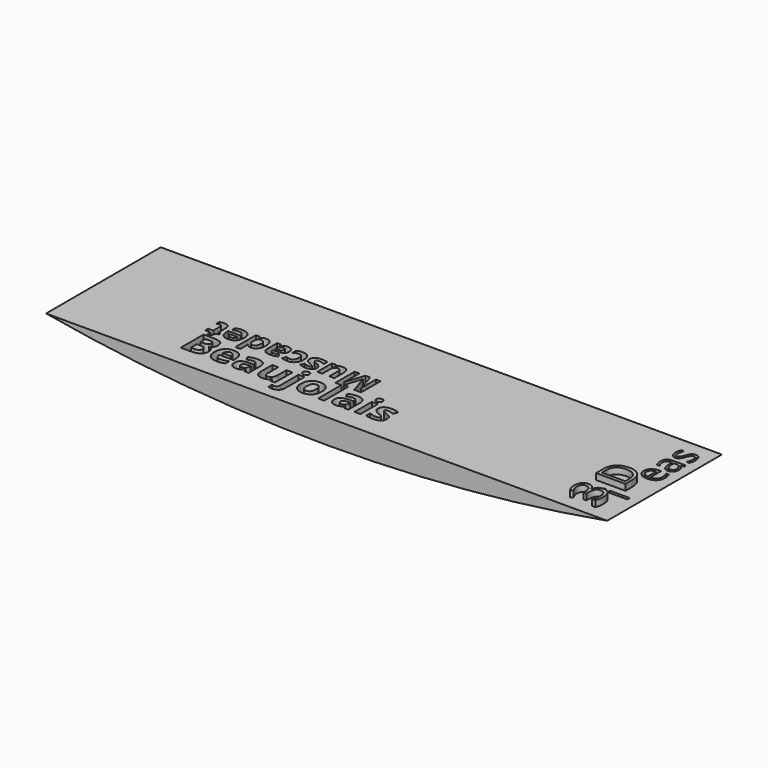
from build123d import *

# Parameters (mm, degrees)
F0_W         = 274
F0_H         = 70
F1_DEPTH     = 12
F2_TEXT_SIZE = 20.006252
F3_DEPTH     = 3
F4_TEXT_SIZE = 18.055556
F5_DEPTH     = 3
F7_DEPTH     = 70.001
F8_W         = 2.90735
F8_H         = 10.659264
F9_DEPTH     = 25


# Not quite as in the source:
# - Text() gives the source's letters only with a copy of the font that has no kerning and outlines rounded to 1/6400 em; it was checked with that copy


with BuildPart() as f1:
    # F0 (on Top) → F1 (new body)
    with BuildSketch(Plane.XY):
        Rectangle(F0_W, F0_H)
    extrude(amount=F1_DEPTH)

    # F2 (on face) → F3 (join)
    with BuildSketch(Plane.XY.offset(12)):
        with Locations(Location((127, -30), (0, 0, 90))):
            Text('3 D', F2_TEXT_SIZE, font='Open Sans', text_align=(TextAlign.LEFT, TextAlign.BOTTOM))
    extrude(amount=F3_DEPTH)

    # F4 (on face) → F5 (cut)
    with BuildSketch(Plane.XY.offset(12)):
        with Locations(Location((132, -18), (0, 0, 90))):
            Text('i   eas', F4_TEXT_SIZE, font='Open Sans', text_align=(TextAlign.LEFT, TextAlign.BOTTOM))
    extrude(amount=-F5_DEPTH, mode=Mode.SUBTRACT)

    # F6 (on face) → F7 (cut, through all)
    with BuildSketch(Plane.XZ.offset(35)):
        with BuildLine():
            ThreePointArc((0, 0), (-68.762272, 3.005732), (-137, 12))
            Line((-137, 12), (-137, 0))
            Line((-137, 0), (0, 0))
        make_face()
        with BuildLine():
            ThreePointArc((137, 12), (68.762272, 3.005732), (0, 0))
            Line((0, 0), (137, 0))
            Line((137, 0), (137, 12))
        make_face()
    extrude(amount=-F7_DEPTH, mode=Mode.SUBTRACT)

    # F8 (on face) → F9 (cut)
    with BuildSketch(Plane.XY.offset(12)):
        with BuildLine():
            Line((-74.907685, -11.061198), (-79.245828, -11.061198))
            Line((-79.245828, -11.061198), (-79.245828, -25))
            Line((-79.245828, -25), (-74.032124, -25))
            add(Edge.make_bspline(
                [(-70.288874, -23.932243), (-71.667806, -25), (-74.032124, -25)],
                knots=[0, 0, 0, 1, 1, 1], degree=2))
            add(Edge.make_bspline(
                [(-68.909942, -20.957778), (-68.909942, -22.864486), (-70.288874, -23.932243)],
                knots=[0, 0, 0, 1, 1, 1], degree=2))
            add(Edge.make_bspline(
                [(-69.497209, -18.802434), (-68.909942, -19.612404), (-68.909942, -20.957778)],
                knots=[0, 0, 0, 1, 1, 1], degree=2))
            add(Edge.make_bspline(
                [(-71.408493, -17.696544), (-70.084475, -17.992465), (-69.497209, -18.802434)],
                knots=[0, 0, 0, 1, 1, 1], degree=2))
            Line((-71.408493, -17.696544), (-71.408493, -17.601971))
            add(Edge.make_bspline(
                [(-69.849568, -16.639464), (-70.435309, -17.440282), (-71.408493, -17.601971)],
                knots=[0, 0, 0, 1, 1, 1], degree=2))
            add(Edge.make_bspline(
                [(-69.263827, -14.587846), (-69.263827, -15.838647), (-69.849568, -16.639464)],
                knots=[0, 0, 0, 1, 1, 1], degree=2))
            add(Edge.make_bspline(
                [(-70.6031, -11.904726), (-69.263827, -12.748253), (-69.263827, -14.587846)],
                knots=[0, 0, 0, 1, 1, 1], degree=2))
            add(Edge.make_bspline(
                [(-74.907685, -11.061198), (-71.942372, -11.061198), (-70.6031, -11.904726)],
                knots=[0, 0, 0, 1, 1, 1], degree=2))
        make_face()
        with BuildLine():
            Line((-76.289667, -22.559413), (-76.289667, -18.925989))
            Line((-76.289667, -18.925989), (-74.459227, -18.925989))
            add(Edge.make_bspline(
                [(-71.982031, -20.661857), (-71.982031, -18.925989), (-74.459227, -18.925989)],
                knots=[0, 0, 0, 1, 1, 1], degree=2))
            add(Edge.make_bspline(
                [(-72.563196, -22.092651), (-71.982031, -21.625889), (-71.982031, -20.661857)],
                knots=[0, 0, 0, 1, 1, 1], degree=2))
            add(Edge.make_bspline(
                [(-74.364654, -22.559413), (-73.144361, -22.559413), (-72.563196, -22.092651)],
                knots=[0, 0, 0, 1, 1, 1], degree=2))
            Line((-74.364654, -22.559413), (-76.289667, -22.559413))
        make_face(mode=Mode.SUBTRACT)
        with BuildLine():
            Line((-74.575155, -16.583026), (-76.289667, -16.583026))
            Line((-76.289667, -16.583026), (-76.289667, -13.48348))
            Line((-76.289667, -13.48348), (-74.736844, -13.48348))
            add(Edge.make_bspline(
                [(-72.881998, -13.831264), (-73.467738, -13.48348), (-74.736844, -13.48348)],
                knots=[0, 0, 0, 1, 1, 1], degree=2))
            add(Edge.make_bspline(
                [(-72.296257, -14.981391), (-72.296257, -14.179048), (-72.881998, -13.831264)],
                knots=[0, 0, 0, 1, 1, 1], degree=2))
            add(Edge.make_bspline(
                [(-72.834711, -16.210836), (-72.296257, -15.838647), (-72.296257, -14.981391)],
                knots=[0, 0, 0, 1, 1, 1], degree=2))
            add(Edge.make_bspline(
                [(-74.575155, -16.583026), (-73.373166, -16.583026), (-72.834711, -16.210836)],
                knots=[0, 0, 0, 1, 1, 1], degree=2))
        make_face(mode=Mode.SUBTRACT)
        with BuildLine():
            add(Edge.make_bspline(
                [(-61.533268, -25.192196), (-64.105037, -25.192196), (-65.554135, -23.770554)],
                knots=[0, 0, 0, 1, 1, 1], degree=2))
            add(Edge.make_bspline(
                [(-59.416059, -25.006101), (-60.282467, -25.192196), (-61.533268, -25.192196)],
                knots=[0, 0, 0, 1, 1, 1], degree=2))
            add(Edge.make_bspline(
                [(-57.786967, -24.438665), (-58.549651, -24.820007), (-59.416059, -25.006101)],
                knots=[0, 0, 0, 1, 1, 1], degree=2))
            Line((-57.786967, -24.438665), (-57.786967, -22.187224))
            add(Edge.make_bspline(
                [(-59.577748, -22.826352), (-58.720492, -22.626529), (-57.786967, -22.187224)],
                knots=[0, 0, 0, 1, 1, 1], degree=2))
            add(Edge.make_bspline(
                [(-61.399036, -23.026175), (-60.435004, -23.026175), (-59.577748, -22.826352)],
                knots=[0, 0, 0, 1, 1, 1], degree=2))
            add(Edge.make_bspline(
                [(-63.324049, -22.330608), (-62.637634, -23.026175), (-61.399036, -23.026175)],
                knots=[0, 0, 0, 1, 1, 1], degree=2))
            add(Edge.make_bspline(
                [(-64.059276, -20.396443), (-64.010464, -21.635041), (-63.324049, -22.330608)],
                knots=[0, 0, 0, 1, 1, 1], degree=2))
            Line((-64.059276, -20.396443), (-57.185973, -20.396443))
            Line((-57.185973, -20.396443), (-57.185973, -18.983953))
            add(Edge.make_bspline(
                [(-58.4444, -15.428323), (-57.185973, -16.714207), (-57.185973, -18.983953)],
                knots=[0, 0, 0, 1, 1, 1], degree=2))
            add(Edge.make_bspline(
                [(-61.960371, -14.142439), (-59.702828, -14.142439), (-58.4444, -15.428323)],
                knots=[0, 0, 0, 1, 1, 1], degree=2))
            add(Edge.make_bspline(
                [(-65.663962, -15.605266), (-64.32469, -14.142439), (-61.960371, -14.142439)],
                knots=[0, 0, 0, 1, 1, 1], degree=2))
            add(Edge.make_bspline(
                [(-67.003234, -19.746637), (-67.003234, -17.068092), (-65.663962, -15.605266)],
                knots=[0, 0, 0, 1, 1, 1], degree=2))
            add(Edge.make_bspline(
                [(-65.554135, -23.770554), (-67.003234, -22.348912), (-67.003234, -19.746637)],
                knots=[0, 0, 0, 1, 1, 1], degree=2))
        make_face()
        with BuildLine():
            add(Edge.make_bspline(
                [(-61.942067, -16.210836), (-62.866439, -16.210836), (-63.391165, -16.796577)],
                knots=[0, 0, 0, 1, 1, 1], degree=2))
            add(Edge.make_bspline(
                [(-60.474664, -16.796577), (-61.017694, -16.210836), (-61.942067, -16.210836)],
                knots=[0, 0, 0, 1, 1, 1], degree=2))
            add(Edge.make_bspline(
                [(-59.910278, -18.459227), (-59.931633, -17.382318), (-60.474664, -16.796577)],
                knots=[0, 0, 0, 1, 1, 1], degree=2))
            Line((-59.910278, -18.459227), (-63.99216, -18.459227))
            add(Edge.make_bspline(
                [(-63.391165, -16.796577), (-63.915891, -17.382318), (-63.99216, -18.459227)],
                knots=[0, 0, 0, 1, 1, 1], degree=2))
        make_face(mode=Mode.SUBTRACT)
        with BuildLine():
            Line((-48.616462, -23.550901), (-48.052076, -25))
            Line((-48.052076, -25), (-46.023338, -25))
            Line((-46.023338, -25), (-46.023338, -17.897892))
            add(Edge.make_bspline(
                [(-47.167363, -15.056134), (-46.023338, -15.991183), (-46.023338, -17.897892)],
                knots=[0, 0, 0, 1, 1, 1], degree=2))
            add(Edge.make_bspline(
                [(-50.456054, -14.121084), (-48.311388, -14.121084), (-47.167363, -15.056134)],
                knots=[0, 0, 0, 1, 1, 1], degree=2))
            add(Edge.make_bspline(
                [(-54.534885, -15.085115), (-52.695293, -14.121084), (-50.456054, -14.121084)],
                knots=[0, 0, 0, 1, 1, 1], degree=2))
            Line((-54.534885, -15.085115), (-53.573904, -17.049788))
            add(Edge.make_bspline(
                [(-50.568931, -16.277952), (-51.847189, -16.277952), (-53.573904, -17.049788)],
                knots=[0, 0, 0, 1, 1, 1], degree=2))
            add(Edge.make_bspline(
                [(-48.909332, -17.897892), (-48.909332, -16.277952), (-50.568931, -16.277952)],
                knots=[0, 0, 0, 1, 1, 1], degree=2))
            Line((-48.909332, -17.897892), (-48.909332, -18.364654))
            Line((-48.909332, -18.364654), (-50.761128, -18.422618))
            add(Edge.make_bspline(
                [(-54.339638, -19.313432), (-53.152903, -18.508039), (-50.761128, -18.422618)],
                knots=[0, 0, 0, 1, 1, 1], degree=2))
            add(Edge.make_bspline(
                [(-55.526374, -21.815034), (-55.526374, -20.118826), (-54.339638, -19.313432)],
                knots=[0, 0, 0, 1, 1, 1], degree=2))
            add(Edge.make_bspline(
                [(-54.644712, -24.313585), (-55.526374, -23.434974), (-55.526374, -21.815034)],
                knots=[0, 0, 0, 1, 1, 1], degree=2))
            add(Edge.make_bspline(
                [(-52.22853, -25.192196), (-53.76305, -25.192196), (-54.644712, -24.313585)],
                knots=[0, 0, 0, 1, 1, 1], degree=2))
            add(Edge.make_bspline(
                [(-50.202843, -24.833735), (-50.98078, -25.192196), (-52.22853, -25.192196)],
                knots=[0, 0, 0, 1, 1, 1], degree=2))
            add(Edge.make_bspline(
                [(-48.69273, -23.550901), (-49.424906, -24.475274), (-50.202843, -24.833735)],
                knots=[0, 0, 0, 1, 1, 1], degree=2))
            Line((-48.69273, -23.550901), (-48.616462, -23.550901))
        make_face()
        with BuildLine():
            Line((-50.035053, -20.100522), (-48.909332, -20.060862))
            Line((-48.909332, -20.060862), (-48.909332, -20.939473))
            add(Edge.make_bspline(
                [(-49.514903, -22.483145), (-48.909332, -21.900455), (-48.909332, -20.939473)],
                knots=[0, 0, 0, 1, 1, 1], degree=2))
            add(Edge.make_bspline(
                [(-51.133317, -23.065835), (-50.120473, -23.065835), (-49.514903, -22.483145)],
                knots=[0, 0, 0, 1, 1, 1], degree=2))
            add(Edge.make_bspline(
                [(-52.542756, -21.833338), (-52.542756, -23.065835), (-51.133317, -23.065835)],
                knots=[0, 0, 0, 1, 1, 1], degree=2))
            add(Edge.make_bspline(
                [(-51.923457, -20.556606), (-52.542756, -20.976082), (-52.542756, -21.833338)],
                knots=[0, 0, 0, 1, 1, 1], degree=2))
            add(Edge.make_bspline(
                [(-50.035053, -20.100522), (-51.304158, -20.13713), (-51.923457, -20.556606)],
                knots=[0, 0, 0, 1, 1, 1], degree=2))
        make_face(mode=Mode.SUBTRACT)
        with BuildLine():
            Line((-35.867446, -23.636322), (-35.476952, -25))
            Line((-35.476952, -25), (-33.246865, -25))
            Line((-33.246865, -25), (-33.246865, -14.340736))
            Line((-33.246865, -14.340736), (-36.154215, -14.340736))
            Line((-36.154215, -14.340736), (-36.154215, -19.356143))
            add(Edge.make_bspline(
                [(-36.697245, -22.059093), (-36.154215, -21.244547), (-36.154215, -19.356143)],
                knots=[0, 0, 0, 1, 1, 1], degree=2))
            add(Edge.make_bspline(
                [(-38.460569, -22.873639), (-37.240276, -22.873639), (-36.697245, -22.059093)],
                knots=[0, 0, 0, 1, 1, 1], degree=2))
            add(Edge.make_bspline(
                [(-39.767809, -22.29705), (-39.357485, -22.873639), (-38.460569, -22.873639)],
                knots=[0, 0, 0, 1, 1, 1], degree=2))
            add(Edge.make_bspline(
                [(-40.178132, -20.567284), (-40.178132, -21.720461), (-39.767809, -22.29705)],
                knots=[0, 0, 0, 1, 1, 1], degree=2))
            Line((-40.178132, -20.567284), (-40.178132, -14.340736))
            Line((-40.178132, -14.340736), (-43.085482, -14.340736))
            Line((-43.085482, -14.340736), (-43.085482, -21.290308))
            add(Edge.make_bspline(
                [(-42.132127, -24.185454), (-43.085482, -23.178712), (-43.085482, -21.290308)],
                knots=[0, 0, 0, 1, 1, 1], degree=2))
            add(Edge.make_bspline(
                [(-39.299521, -25.192196), (-41.178773, -25.192196), (-42.132127, -24.185454)],
                knots=[0, 0, 0, 1, 1, 1], degree=2))
            add(Edge.make_bspline(
                [(-37.345526, -24.786449), (-38.204308, -25.192196), (-39.299521, -25.192196)],
                knots=[0, 0, 0, 1, 1, 1], degree=2))
            add(Edge.make_bspline(
                [(-36.019982, -23.636322), (-36.486745, -24.380701), (-37.345526, -24.786449)],
                knots=[0, 0, 0, 1, 1, 1], degree=2))
            Line((-36.019982, -23.636322), (-35.867446, -23.636322))
        make_face()
        with BuildLine():
            add(Edge.make_bspline(
                [(-31.053388, -29.692028), (-32.169956, -29.692028), (-32.969249, -29.45102)],
                knots=[0, 0, 0, 1, 1, 1], degree=2))
            add(Edge.make_bspline(
                [(-28.271119, -28.770707), (-29.253455, -29.692028), (-31.053388, -29.692028)],
                knots=[0, 0, 0, 1, 1, 1], degree=2))
            add(Edge.make_bspline(
                [(-27.288782, -26.153177), (-27.288782, -27.849385), (-28.271119, -28.770707)],
                knots=[0, 0, 0, 1, 1, 1], degree=2))
            Line((-27.288782, -26.153177), (-27.288782, -14.340736))
            Line((-27.288782, -14.340736), (-30.196132, -14.340736))
            Line((-30.196132, -14.340736), (-30.196132, -25.726075))
            add(Edge.make_bspline(
                [(-30.534763, -26.935691), (-30.196132, -26.525367), (-30.196132, -25.726075)],
                knots=[0, 0, 0, 1, 1, 1], degree=2))
            add(Edge.make_bspline(
                [(-31.605571, -27.346014), (-30.873395, -27.346014), (-30.534763, -26.935691)],
                knots=[0, 0, 0, 1, 1, 1], degree=2))
            add(Edge.make_bspline(
                [(-32.969249, -27.16297), (-32.304189, -27.346014), (-31.605571, -27.346014)],
                knots=[0, 0, 0, 1, 1, 1], degree=2))
            Line((-32.969249, -27.16297), (-32.969249, -29.45102))
        make_face()
        with BuildLine():
            add(Edge.make_bspline(
                [(-30.321212, -11.585924), (-30.321212, -10.164282), (-28.737881, -10.164282)],
                knots=[0, 0, 0, 1, 1, 1], degree=2))
            add(Edge.make_bspline(
                [(-28.737881, -13.016718), (-30.321212, -13.016718), (-30.321212, -11.585924)],
                knots=[0, 0, 0, 1, 1, 1], degree=2))
            add(Edge.make_bspline(
                [(-27.54962, -12.639952), (-27.94469, -13.016718), (-28.737881, -13.016718)],
                knots=[0, 0, 0, 1, 1, 1], degree=2))
            add(Edge.make_bspline(
                [(-27.15455, -11.585924), (-27.15455, -12.263187), (-27.54962, -12.639952)],
                knots=[0, 0, 0, 1, 1, 1], degree=2))
            add(Edge.make_bspline(
                [(-28.737881, -10.164282), (-27.15455, -10.164282), (-27.15455, -11.585924)],
                knots=[0, 0, 0, 1, 1, 1], degree=2))
        make_face()
        with BuildLine():
            add(Edge.make_bspline(
                [(-14.551969, -19.652064), (-14.551969, -22.25434), (-15.924799, -23.723268)],
                knots=[0, 0, 0, 1, 1, 1], degree=2))
            add(Edge.make_bspline(
                [(-15.18042, -16.724885), (-14.551969, -17.97416), (-14.551969, -19.652064)],
                knots=[0, 0, 0, 1, 1, 1], degree=2))
            add(Edge.make_bspline(
                [(-16.981879, -14.809024), (-15.808872, -15.475609), (-15.18042, -16.724885)],
                knots=[0, 0, 0, 1, 1, 1], degree=2))
            add(Edge.make_bspline(
                [(-19.689405, -14.142439), (-18.154886, -14.142439), (-16.981879, -14.809024)],
                knots=[0, 0, 0, 1, 1, 1], degree=2))
            add(Edge.make_bspline(
                [(-23.522652, -15.591537), (-22.160499, -14.142439), (-19.689405, -14.142439)],
                knots=[0, 0, 0, 1, 1, 1], degree=2))
            add(Edge.make_bspline(
                [(-24.884804, -19.652064), (-24.884804, -17.040636), (-23.522652, -15.591537)],
                knots=[0, 0, 0, 1, 1, 1], degree=2))
            add(Edge.make_bspline(
                [(-24.256353, -22.588395), (-24.884804, -21.329967), (-24.884804, -19.652064)],
                knots=[0, 0, 0, 1, 1, 1], degree=2))
            add(Edge.make_bspline(
                [(-22.454895, -24.519509), (-23.627902, -23.846823), (-24.256353, -22.588395)],
                knots=[0, 0, 0, 1, 1, 1], degree=2))
            add(Edge.make_bspline(
                [(-19.747369, -25.192196), (-21.281888, -25.192196), (-22.454895, -24.519509)],
                knots=[0, 0, 0, 1, 1, 1], degree=2))
            add(Edge.make_bspline(
                [(-15.924799, -23.723268), (-17.29763, -25.192196), (-19.747369, -25.192196)],
                knots=[0, 0, 0, 1, 1, 1], degree=2))
        make_face()
        with BuildLine():
            add(Edge.make_bspline(
                [(-21.922542, -19.652064), (-21.922542, -21.235395), (-21.402392, -22.045364)],
                knots=[0, 0, 0, 1, 1, 1], degree=2))
            add(Edge.make_bspline(
                [(-21.406968, -17.272492), (-21.922542, -18.059581), (-21.922542, -19.652064)],
                knots=[0, 0, 0, 1, 1, 1], degree=2))
            add(Edge.make_bspline(
                [(-19.729064, -16.485402), (-20.891394, -16.485402), (-21.406968, -17.272492)],
                knots=[0, 0, 0, 1, 1, 1], degree=2))
            add(Edge.make_bspline(
                [(-18.040483, -17.277068), (-18.554532, -16.485402), (-19.729064, -16.485402)],
                knots=[0, 0, 0, 1, 1, 1], degree=2))
            add(Edge.make_bspline(
                [(-17.526435, -19.652064), (-17.526435, -18.068733), (-18.040483, -17.277068)],
                knots=[0, 0, 0, 1, 1, 1], degree=2))
            add(Edge.make_bspline(
                [(-18.035907, -22.049941), (-17.526435, -21.244547), (-17.526435, -19.652064)],
                knots=[0, 0, 0, 1, 1, 1], degree=2))
            add(Edge.make_bspline(
                [(-19.71076, -22.855334), (-18.54538, -22.855334), (-18.035907, -22.049941)],
                knots=[0, 0, 0, 1, 1, 1], degree=2))
            add(Edge.make_bspline(
                [(-21.402392, -22.045364), (-20.882242, -22.855334), (-19.71076, -22.855334)],
                knots=[0, 0, 0, 1, 1, 1], degree=2))
        make_face(mode=Mode.SUBTRACT)
        Polygon((-12.147991, -25), (-9.240642, -25), (-9.240642, -10.164282), (-11.470686, -10.164282), (-11.693005, -10.841512), (-12.147991, -10.841512), align=None)
        with BuildLine():
            Line((-15.096382, -10.841512), (-12.147991, -10.841512))
            Line((-12.147991, -10.841512), (-12.147991, -10.164282))
            Line((-12.147991, -10.164282), (-11.470686, -10.164282))
            Line((-11.470686, -10.164282), (-8.73119, -1.819208))
            Line((-8.73119, -1.819208), (-8.682128, -1.819208))
            Line((-8.682128, -1.819208), (-5.890739, -10.841512))
            Line((-5.890739, -10.841512), (-2.484781, -10.841512))
            Line((-2.484781, -10.841512), (-2.484781, 0.956687))
            Line((-2.484781, 0.956687), (-4.72099, 0.956687))
            Line((-4.72099, 0.956687), (-4.72099, -4.530547))
            add(Edge.make_bspline(
                [(-4.566057, -8.298018), (-4.72099, -5.475643), (-4.72099, -4.530547)],
                knots=[0, 0, 0, 1, 1, 1], degree=2))
            Line((-4.566057, -8.298018), (-4.638359, -8.298018))
            Line((-4.638359, -8.298018), (-7.47881, 0.956687))
            Line((-7.47881, 0.956687), (-9.771828, 0.956687))
            Line((-9.771828, 0.956687), (-12.813692, -8.282524))
            Line((-12.813692, -8.282524), (-12.885995, -8.282524))
            add(Edge.make_bspline(
                [(-12.777541, -5.540199), (-12.790452, -6.056644), (-12.885995, -8.282524)],
                knots=[0, 0, 0, 1, 1, 1], degree=2))
            add(Edge.make_bspline(
                [(-12.76463, -4.628672), (-12.76463, -5.023753), (-12.777541, -5.540199)],
                knots=[0, 0, 0, 1, 1, 1], degree=2))
            Line((-12.76463, -4.628672), (-12.76463, 0.956687))
            Line((-12.76463, 0.956687), (-15.096382, 0.956687))
            Line((-15.096382, 0.956687), (-15.096382, -10.841512))
        make_face()
        Polygon((-12.147991, -10.164282), (-12.147991, -10.841512), (-11.693005, -10.841512), (-11.470686, -10.164282), align=None)
        with BuildLine():
            Line((0.015284, -23.550901), (0.57967, -25))
            Line((0.57967, -25), (2.608408, -25))
            Line((2.608408, -25), (2.608408, -17.897892))
            add(Edge.make_bspline(
                [(1.464383, -15.056134), (2.608408, -15.991183), (2.608408, -17.897892)],
                knots=[0, 0, 0, 1, 1, 1], degree=2))
            add(Edge.make_bspline(
                [(-1.824308, -14.121084), (0.320358, -14.121084), (1.464383, -15.056134)],
                knots=[0, 0, 0, 1, 1, 1], degree=2))
            add(Edge.make_bspline(
                [(-5.903139, -15.085115), (-4.063547, -14.121084), (-1.824308, -14.121084)],
                knots=[0, 0, 0, 1, 1, 1], degree=2))
            Line((-5.903139, -15.085115), (-4.942158, -17.049788))
            add(Edge.make_bspline(
                [(-1.937185, -16.277952), (-3.215443, -16.277952), (-4.942158, -17.049788)],
                knots=[0, 0, 0, 1, 1, 1], degree=2))
            add(Edge.make_bspline(
                [(-0.277586, -17.897892), (-0.277586, -16.277952), (-1.937185, -16.277952)],
                knots=[0, 0, 0, 1, 1, 1], degree=2))
            Line((-0.277586, -17.897892), (-0.277586, -18.364654))
            Line((-0.277586, -18.364654), (-2.129382, -18.422618))
            add(Edge.make_bspline(
                [(-5.707892, -19.313432), (-4.521157, -18.508039), (-2.129382, -18.422618)],
                knots=[0, 0, 0, 1, 1, 1], degree=2))
            add(Edge.make_bspline(
                [(-6.894628, -21.815034), (-6.894628, -20.118826), (-5.707892, -19.313432)],
                knots=[0, 0, 0, 1, 1, 1], degree=2))
            add(Edge.make_bspline(
                [(-6.012966, -24.313585), (-6.894628, -23.434974), (-6.894628, -21.815034)],
                knots=[0, 0, 0, 1, 1, 1], degree=2))
            add(Edge.make_bspline(
                [(-3.596785, -25.192196), (-5.131304, -25.192196), (-6.012966, -24.313585)],
                knots=[0, 0, 0, 1, 1, 1], degree=2))
            add(Edge.make_bspline(
                [(-1.571097, -24.833735), (-2.349034, -25.192196), (-3.596785, -25.192196)],
                knots=[0, 0, 0, 1, 1, 1], degree=2))
            add(Edge.make_bspline(
                [(-0.060984, -23.550901), (-0.79316, -24.475274), (-1.571097, -24.833735)],
                knots=[0, 0, 0, 1, 1, 1], degree=2))
            Line((-0.060984, -23.550901), (0.015284, -23.550901))
        make_face()
        with BuildLine():
            Line((-1.403307, -20.100522), (-0.277586, -20.060862))
            Line((-0.277586, -20.060862), (-0.277586, -20.939473))
            add(Edge.make_bspline(
                [(-0.883157, -22.483145), (-0.277586, -21.900455), (-0.277586, -20.939473)],
                knots=[0, 0, 0, 1, 1, 1], degree=2))
            add(Edge.make_bspline(
                [(-2.501571, -23.065835), (-1.488728, -23.065835), (-0.883157, -22.483145)],
                knots=[0, 0, 0, 1, 1, 1], degree=2))
            add(Edge.make_bspline(
                [(-3.91101, -21.833338), (-3.91101, -23.065835), (-2.501571, -23.065835)],
                knots=[0, 0, 0, 1, 1, 1], degree=2))
            add(Edge.make_bspline(
                [(-3.291711, -20.556606), (-3.91101, -20.976082), (-3.91101, -21.833338)],
                knots=[0, 0, 0, 1, 1, 1], degree=2))
            add(Edge.make_bspline(
                [(-1.403307, -20.100522), (-2.672412, -20.13713), (-3.291711, -20.556606)],
                knots=[0, 0, 0, 1, 1, 1], degree=2))
        make_face(mode=Mode.SUBTRACT)
        with BuildLine():
            add(Edge.make_bspline(
                [(5.479148, -11.585924), (5.479148, -10.164282), (7.062479, -10.164282)],
                knots=[0, 0, 0, 1, 1, 1], degree=2))
            add(Edge.make_bspline(
                [(7.062479, -13.016718), (5.479148, -13.016718), (5.479148, -11.585924)],
                knots=[0, 0, 0, 1, 1, 1], degree=2))
            add(Edge.make_bspline(
                [(8.25074, -12.639952), (7.85567, -13.016718), (7.062479, -13.016718)],
                knots=[0, 0, 0, 1, 1, 1], degree=2))
            add(Edge.make_bspline(
                [(8.64581, -11.585924), (8.64581, -12.263187), (8.25074, -12.639952)],
                knots=[0, 0, 0, 1, 1, 1], degree=2))
            add(Edge.make_bspline(
                [(7.062479, -10.164282), (8.64581, -10.164282), (8.64581, -11.585924)],
                knots=[0, 0, 0, 1, 1, 1], degree=2))
        make_face()
        with Locations((7.057903, -19.670368)):
            Rectangle(F8_W, F8_H)
        with BuildLine():
            add(Edge.make_bspline(
                [(19, -21.833338), (19, -23.474633), (17.860551, -24.333415)],
                knots=[0, 0, 0, 1, 1, 1], degree=2))
            add(Edge.make_bspline(
                [(18.722383, -20.471186), (19, -21.043198), (19, -21.833338)],
                knots=[0, 0, 0, 1, 1, 1], degree=2))
            add(Edge.make_bspline(
                [(17.863602, -19.461393), (18.444766, -19.899173), (18.722383, -20.471186)],
                knots=[0, 0, 0, 1, 1, 1], degree=2))
            add(Edge.make_bspline(
                [(16.034687, -18.517191), (17.282437, -19.023613), (17.863602, -19.461393)],
                knots=[0, 0, 0, 1, 1, 1], degree=2))
            add(Edge.make_bspline(
                [(14.21645, -17.669087), (14.631349, -17.955856), (16.034687, -18.517191)],
                knots=[0, 0, 0, 1, 1, 1], degree=2))
            add(Edge.make_bspline(
                [(13.80155, -16.991824), (13.80155, -17.382318), (14.21645, -17.669087)],
                knots=[0, 0, 0, 1, 1, 1], degree=2))
            add(Edge.make_bspline(
                [(15.088959, -16.296257), (13.80155, -16.296257), (13.80155, -16.991824)],
                knots=[0, 0, 0, 1, 1, 1], degree=2))
            add(Edge.make_bspline(
                [(16.510601, -16.51591), (15.815034, -16.296257), (15.088959, -16.296257)],
                knots=[0, 0, 0, 1, 1, 1], degree=2))
            add(Edge.make_bspline(
                [(18.008512, -17.077245), (17.206169, -16.735562), (16.510601, -16.51591)],
                knots=[0, 0, 0, 1, 1, 1], degree=2))
            Line((18.008512, -17.077245), (18.884072, -14.981391))
            add(Edge.make_bspline(
                [(15.137771, -14.142439), (17.062784, -14.142439), (18.884072, -14.981391)],
                knots=[0, 0, 0, 1, 1, 1], degree=2))
            add(Edge.make_bspline(
                [(12.015345, -14.91885), (13.115135, -14.142439), (15.137771, -14.142439)],
                knots=[0, 0, 0, 1, 1, 1], degree=2))
            add(Edge.make_bspline(
                [(10.915556, -17.116904), (10.915556, -15.695262), (12.015345, -14.91885)],
                knots=[0, 0, 0, 1, 1, 1], degree=2))
            add(Edge.make_bspline(
                [(11.176393, -18.511089), (10.915556, -17.943653), (10.915556, -17.116904)],
                knots=[0, 0, 0, 1, 1, 1], degree=2))
            add(Edge.make_bspline(
                [(12.015345, -19.517832), (11.437231, -19.078526), (11.176393, -18.511089)],
                knots=[0, 0, 0, 1, 1, 1], degree=2))
            add(Edge.make_bspline(
                [(13.822905, -20.472711), (12.593459, -19.957137), (12.015345, -19.517832)],
                knots=[0, 0, 0, 1, 1, 1], degree=2))
            add(Edge.make_bspline(
                [(15.19421, -21.104213), (14.680161, -20.832698), (13.822905, -20.472711)],
                knots=[0, 0, 0, 1, 1, 1], degree=2))
            add(Edge.make_bspline(
                [(15.918759, -21.590805), (15.708258, -21.375728), (15.19421, -21.104213)],
                knots=[0, 0, 0, 1, 1, 1], degree=2))
            add(Edge.make_bspline(
                [(16.12926, -22.150615), (16.12926, -21.805882), (15.918759, -21.590805)],
                knots=[0, 0, 0, 1, 1, 1], degree=2))
            add(Edge.make_bspline(
                [(14.545929, -23.065835), (16.12926, -23.065835), (16.12926, -22.150615)],
                knots=[0, 0, 0, 1, 1, 1], degree=2))
            add(Edge.make_bspline(
                [(12.758199, -22.808048), (13.774093, -23.065835), (14.545929, -23.065835)],
                knots=[0, 0, 0, 1, 1, 1], degree=2))
            add(Edge.make_bspline(
                [(10.93386, -22.168919), (11.742305, -22.550261), (12.758199, -22.808048)],
                knots=[0, 0, 0, 1, 1, 1], degree=2))
            Line((10.93386, -22.168919), (10.93386, -24.569847))
            add(Edge.make_bspline(
                [(12.468379, -25.033558), (11.647732, -24.87492), (10.93386, -24.569847)],
                knots=[0, 0, 0, 1, 1, 1], degree=2))
            add(Edge.make_bspline(
                [(14.451356, -25.192196), (13.289027, -25.192196), (12.468379, -25.033558)],
                knots=[0, 0, 0, 1, 1, 1], degree=2))
            add(Edge.make_bspline(
                [(17.860551, -24.333415), (16.721102, -25.192196), (14.451356, -25.192196)],
                knots=[0, 0, 0, 1, 1, 1], degree=2))
        make_face()
        with BuildLine():
            Line((-23.932765, -0.197569), (-24.26329, 0.956687))
            Line((-24.26329, 0.956687), (-26.150899, 0.956687))
            Line((-26.150899, 0.956687), (-26.150899, -8.065617))
            Line((-26.150899, -8.065617), (-23.690036, -8.065617))
            Line((-23.690036, -8.065617), (-23.690036, -3.820435))
            add(Edge.make_bspline(
                [(-23.230399, -1.532581), (-23.690036, -2.222036), (-23.690036, -3.820435)],
                knots=[0, 0, 0, 1, 1, 1], degree=2))
            add(Edge.make_bspline(
                [(-21.737872, -0.843126), (-22.770763, -0.843126), (-23.230399, -1.532581)],
                knots=[0, 0, 0, 1, 1, 1], degree=2))
            add(Edge.make_bspline(
                [(-20.631387, -1.331167), (-20.978697, -0.843126), (-21.737872, -0.843126)],
                knots=[0, 0, 0, 1, 1, 1], degree=2))
            add(Edge.make_bspline(
                [(-20.284077, -2.79529), (-20.284077, -1.819208), (-20.631387, -1.331167)],
                knots=[0, 0, 0, 1, 1, 1], degree=2))
            Line((-20.284077, -2.79529), (-20.284077, -8.065617))
            Line((-20.284077, -8.065617), (-17.823214, -8.065617))
            Line((-17.823214, -8.065617), (-17.823214, -2.183302))
            add(Edge.make_bspline(
                [(-18.63016, 0.267232), (-17.823214, -0.584903), (-17.823214, -2.183302)],
                knots=[0, 0, 0, 1, 1, 1], degree=2))
            add(Edge.make_bspline(
                [(-21.027759, 1.119367), (-19.437107, 1.119367), (-18.63016, 0.267232)],
                knots=[0, 0, 0, 1, 1, 1], degree=2))
            add(Edge.make_bspline(
                [(-22.681676, 0.775931), (-21.954779, 1.119367), (-21.027759, 1.119367)],
                knots=[0, 0, 0, 1, 1, 1], degree=2))
            add(Edge.make_bspline(
                [(-23.803654, -0.197569), (-23.408573, 0.432494), (-22.681676, 0.775931)],
                knots=[0, 0, 0, 1, 1, 1], degree=2))
            Line((-23.803654, -0.197569), (-23.932765, -0.197569))
        make_face()
        with BuildLine():
            add(Edge.make_bspline(
                [(-35.028598, -1.723666), (-35.028598, -0.334427), (-34.064136, 0.39247)],
                knots=[0, 0, 0, 1, 1, 1], degree=2))
            add(Edge.make_bspline(
                [(-34.793615, -2.876631), (-35.028598, -2.392463), (-35.028598, -1.723666)],
                knots=[0, 0, 0, 1, 1, 1], degree=2))
            add(Edge.make_bspline(
                [(-34.066718, -3.731348), (-34.558633, -3.360798), (-34.793615, -2.876631)],
                knots=[0, 0, 0, 1, 1, 1], degree=2))
            add(Edge.make_bspline(
                [(-32.518673, -4.530547), (-33.574804, -4.101898), (-34.066718, -3.731348)],
                knots=[0, 0, 0, 1, 1, 1], degree=2))
            add(Edge.make_bspline(
                [(-30.979665, -5.248407), (-31.330848, -5.005677), (-32.518673, -4.530547)],
                knots=[0, 0, 0, 1, 1, 1], degree=2))
            add(Edge.make_bspline(
                [(-30.628482, -5.821661), (-30.628482, -5.491136), (-30.979665, -5.248407)],
                knots=[0, 0, 0, 1, 1, 1], degree=2))
            add(Edge.make_bspline(
                [(-31.718182, -6.410409), (-30.628482, -6.410409), (-30.628482, -5.821661)],
                knots=[0, 0, 0, 1, 1, 1], degree=2))
            add(Edge.make_bspline(
                [(-32.9215, -6.224489), (-32.332752, -6.410409), (-31.718182, -6.410409)],
                knots=[0, 0, 0, 1, 1, 1], degree=2))
            add(Edge.make_bspline(
                [(-34.189374, -5.749359), (-33.510248, -6.038568), (-32.9215, -6.224489)],
                knots=[0, 0, 0, 1, 1, 1], degree=2))
            Line((-34.189374, -5.749359), (-34.930474, -7.523349))
            add(Edge.make_bspline(
                [(-31.759498, -8.233462), (-33.388884, -8.233462), (-34.930474, -7.523349)],
                knots=[0, 0, 0, 1, 1, 1], degree=2))
            add(Edge.make_bspline(
                [(-29.116588, -7.576285), (-30.047481, -8.233462), (-31.759498, -8.233462)],
                knots=[0, 0, 0, 1, 1, 1], degree=2))
            add(Edge.make_bspline(
                [(-28.185694, -5.71579), (-28.185694, -6.919108), (-29.116588, -7.576285)],
                knots=[0, 0, 0, 1, 1, 1], degree=2))
            add(Edge.make_bspline(
                [(-28.406475, -4.535712), (-28.185694, -5.016006), (-28.185694, -5.71579)],
                knots=[0, 0, 0, 1, 1, 1], degree=2))
            add(Edge.make_bspline(
                [(-29.116588, -3.683577), (-28.627255, -4.055418), (-28.406475, -4.535712)],
                knots=[0, 0, 0, 1, 1, 1], degree=2))
            add(Edge.make_bspline(
                [(-30.646558, -2.875339), (-29.60592, -3.311736), (-29.116588, -3.683577)],
                knots=[0, 0, 0, 1, 1, 1], degree=2))
            add(Edge.make_bspline(
                [(-31.807269, -2.340818), (-31.372164, -2.570637), (-30.646558, -2.875339)],
                knots=[0, 0, 0, 1, 1, 1], degree=2))
            add(Edge.make_bspline(
                [(-32.420548, -1.928953), (-32.242374, -2.111), (-31.807269, -2.340818)],
                knots=[0, 0, 0, 1, 1, 1], degree=2))
            add(Edge.make_bspline(
                [(-32.598722, -1.455114), (-32.598722, -1.746906), (-32.420548, -1.928953)],
                knots=[0, 0, 0, 1, 1, 1], degree=2))
            add(Edge.make_bspline(
                [(-31.258546, -0.680446), (-32.598722, -0.680446), (-32.598722, -1.455114)],
                knots=[0, 0, 0, 1, 1, 1], degree=2))
            add(Edge.make_bspline(
                [(-29.74536, -0.898644), (-30.605242, -0.680446), (-31.258546, -0.680446)],
                knots=[0, 0, 0, 1, 1, 1], degree=2))
            add(Edge.make_bspline(
                [(-28.201188, -1.439621), (-28.885478, -1.116842), (-29.74536, -0.898644)],
                knots=[0, 0, 0, 1, 1, 1], degree=2))
            Line((-28.201188, -1.439621), (-28.201188, 0.592593))
            add(Edge.make_bspline(
                [(-29.500048, 0.985091), (-28.805429, 0.850815), (-28.201188, 0.592593)],
                knots=[0, 0, 0, 1, 1, 1], degree=2))
            add(Edge.make_bspline(
                [(-31.178496, 1.119367), (-30.194668, 1.119367), (-29.500048, 0.985091)],
                knots=[0, 0, 0, 1, 1, 1], degree=2))
            add(Edge.make_bspline(
                [(-34.064136, 0.39247), (-33.099674, 1.119367), (-31.178496, 1.119367)],
                knots=[0, 0, 0, 1, 1, 1], degree=2))
        make_face()
        with BuildLine():
            add(Edge.make_bspline(
                [(-40.611375, 1.119367), (-36.399761, 1.119367), (-36.399761, -3.505403)],
                knots=[0, 0, 0, 1, 1, 1], degree=2))
            add(Edge.make_bspline(
                [(-42.1478, 0.973471), (-41.538394, 1.119367), (-40.611375, 1.119367)],
                knots=[0, 0, 0, 1, 1, 1], degree=2))
            add(Edge.make_bspline(
                [(-43.353701, 0.447988), (-42.757206, 0.827575), (-42.1478, 0.973471)],
                knots=[0, 0, 0, 1, 1, 1], degree=2))
            Line((-43.353701, 0.447988), (-43.353701, -1.65911))
            add(Edge.make_bspline(
                [(-42.143927, -1.063907), (-42.749459, -1.2537), (-43.353701, -1.65911)],
                knots=[0, 0, 0, 1, 1, 1], degree=2))
            add(Edge.make_bspline(
                [(-40.828282, -0.874113), (-41.538394, -0.874113), (-42.143927, -1.063907)],
                knots=[0, 0, 0, 1, 1, 1], degree=2))
            add(Edge.make_bspline(
                [(-38.907104, -3.520896), (-38.907104, -0.874113), (-40.828282, -0.874113)],
                knots=[0, 0, 0, 1, 1, 1], degree=2))
            add(Edge.make_bspline(
                [(-40.828282, -6.250311), (-38.907104, -6.250311), (-38.907104, -3.520896)],
                knots=[0, 0, 0, 1, 1, 1], degree=2))
            add(Edge.make_bspline(
                [(-41.828895, -6.100542), (-41.329234, -6.250311), (-40.828282, -6.250311)],
                knots=[0, 0, 0, 1, 1, 1], degree=2))
            add(Edge.make_bspline(
                [(-42.909557, -5.71579), (-42.328556, -5.950773), (-41.828895, -6.100542)],
                knots=[0, 0, 0, 1, 1, 1], degree=2))
            Line((-42.909557, -5.71579), (-43.637746, -7.621474))
            add(Edge.make_bspline(
                [(-40.828282, -8.233462), (-42.393112, -8.233462), (-43.637746, -7.621474)],
                knots=[0, 0, 0, 1, 1, 1], degree=2))
            add(Edge.make_bspline(
                [(-37.544979, -7.019815), (-38.690197, -8.233462), (-40.828282, -8.233462)],
                knots=[0, 0, 0, 1, 1, 1], degree=2))
            add(Edge.make_bspline(
                [(-36.399761, -3.505403), (-36.399761, -5.806168), (-37.544979, -7.019815)],
                knots=[0, 0, 0, 1, 1, 1], degree=2))
        make_face()
        with BuildLine():
            Line((-50.697557, -0.269872), (-51.175269, 0.956687))
            Line((-51.175269, 0.956687), (-52.89245, 0.956687))
            Line((-52.89245, 0.956687), (-52.89245, -5.05474))
            add(Edge.make_bspline(
                [(-51.924115, -7.460085), (-52.89245, -6.668632), (-52.89245, -5.05474)],
                knots=[0, 0, 0, 1, 1, 1], degree=2))
            add(Edge.make_bspline(
                [(-49.140473, -8.251538), (-50.955779, -8.251538), (-51.924115, -7.460085)],
                knots=[0, 0, 0, 1, 1, 1], degree=2))
            add(Edge.make_bspline(
                [(-45.688035, -7.435554), (-47.245118, -8.251538), (-49.140473, -8.251538)],
                knots=[0, 0, 0, 1, 1, 1], degree=2))
            Line((-45.688035, -7.435554), (-46.501436, -5.772599))
            add(Edge.make_bspline(
                [(-49.044931, -6.425903), (-47.962977, -6.425903), (-46.501436, -5.772599)],
                knots=[0, 0, 0, 1, 1, 1], degree=2))
            add(Edge.make_bspline(
                [(-50.449663, -5.05474), (-50.449663, -6.425903), (-49.044931, -6.425903)],
                knots=[0, 0, 0, 1, 1, 1], degree=2))
            Line((-50.449663, -5.05474), (-50.449663, -4.659659))
            Line((-50.449663, -4.659659), (-48.88225, -4.610596))
            add(Edge.make_bspline(
                [(-45.853297, -3.856586), (-46.857784, -4.538294), (-48.88225, -4.610596)],
                knots=[0, 0, 0, 1, 1, 1], degree=2))
            add(Edge.make_bspline(
                [(-44.848811, -1.739159), (-44.848811, -3.174878), (-45.853297, -3.856586)],
                knots=[0, 0, 0, 1, 1, 1], degree=2))
            add(Edge.make_bspline(
                [(-45.595074, 0.375685), (-44.848811, -0.367996), (-44.848811, -1.739159)],
                knots=[0, 0, 0, 1, 1, 1], degree=2))
            add(Edge.make_bspline(
                [(-47.640199, 1.119367), (-46.341338, 1.119367), (-45.595074, 0.375685)],
                knots=[0, 0, 0, 1, 1, 1], degree=2))
            add(Edge.make_bspline(
                [(-49.354798, 0.815955), (-48.69633, 1.119367), (-47.640199, 1.119367)],
                knots=[0, 0, 0, 1, 1, 1], degree=2))
            add(Edge.make_bspline(
                [(-50.633001, -0.269872), (-50.013266, 0.512543), (-49.354798, 0.815955)],
                knots=[0, 0, 0, 1, 1, 1], degree=2))
            Line((-50.633001, -0.269872), (-50.697557, -0.269872))
        make_face()
        with BuildLine():
            Line((-49.496821, -3.190371), (-50.449663, -3.22394))
            Line((-50.449663, -3.22394), (-50.449663, -2.480259))
            add(Edge.make_bspline(
                [(-49.93709, -1.173651), (-50.449663, -1.666857), (-50.449663, -2.480259)],
                knots=[0, 0, 0, 1, 1, 1], degree=2))
            add(Edge.make_bspline(
                [(-48.567219, -0.680446), (-49.424518, -0.680446), (-49.93709, -1.173651)],
                knots=[0, 0, 0, 1, 1, 1], degree=2))
            add(Edge.make_bspline(
                [(-47.374229, -1.723666), (-47.374229, -0.680446), (-48.567219, -0.680446)],
                knots=[0, 0, 0, 1, 1, 1], degree=2))
            add(Edge.make_bspline(
                [(-47.898422, -2.804328), (-47.374229, -2.449272), (-47.374229, -1.723666)],
                knots=[0, 0, 0, 1, 1, 1], degree=2))
            add(Edge.make_bspline(
                [(-49.496821, -3.190371), (-48.422614, -3.159384), (-47.898422, -2.804328)],
                knots=[0, 0, 0, 1, 1, 1], degree=2))
        make_face(mode=Mode.SUBTRACT)
        with BuildLine():
            add(Edge.make_bspline(
                [(-58.284142, 1.119367), (-56.696072, 1.119367), (-55.788419, -0.116229)],
                knots=[0, 0, 0, 1, 1, 1], degree=2))
            add(Edge.make_bspline(
                [(-60.84313, -0.213063), (-60.003906, 1.119367), (-58.284142, 1.119367)],
                knots=[0, 0, 0, 1, 1, 1], degree=2))
            Line((-60.84313, -0.213063), (-60.949001, -0.213063))
            Line((-60.949001, -0.213063), (-61.424131, 0.956687))
            Line((-61.424131, 0.956687), (-63.311739, 0.956687))
            Line((-63.311739, 0.956687), (-63.311739, -11.600687))
            Line((-63.311739, -11.600687), (-60.84313, -11.600687))
            Line((-60.84313, -11.600687), (-60.84313, -8.711174))
            add(Edge.make_bspline(
                [(-61.02905, -6.911361), (-60.84313, -7.921013), (-60.84313, -8.711174)],
                knots=[0, 0, 0, 1, 1, 1], degree=2))
            Line((-61.02905, -6.911361), (-60.949001, -6.911361))
            add(Edge.make_bspline(
                [(-58.348698, -8.233462), (-60.052968, -8.233462), (-60.949001, -6.911361)],
                knots=[0, 0, 0, 1, 1, 1], degree=2))
            add(Edge.make_bspline(
                [(-55.803912, -6.995284), (-56.727059, -8.233462), (-58.348698, -8.233462)],
                knots=[0, 0, 0, 1, 1, 1], degree=2))
            add(Edge.make_bspline(
                [(-54.880766, -3.538972), (-54.880766, -5.757106), (-55.803912, -6.995284)],
                knots=[0, 0, 0, 1, 1, 1], degree=2))
            add(Edge.make_bspline(
                [(-55.788419, -0.116229), (-54.880766, -1.351825), (-54.880766, -3.538972)],
                knots=[0, 0, 0, 1, 1, 1], degree=2))
        make_face()
        with BuildLine():
            add(Edge.make_bspline(
                [(-59.149188, -0.843126), (-60.091701, -0.843126), (-60.531971, -1.39185)],
                knots=[0, 0, 0, 1, 1, 1], degree=2))
            add(Edge.make_bspline(
                [(-57.832252, -1.509341), (-58.291889, -0.843126), (-59.149188, -0.843126)],
                knots=[0, 0, 0, 1, 1, 1], degree=2))
            add(Edge.make_bspline(
                [(-57.372615, -3.505403), (-57.372615, -2.175556), (-57.832252, -1.509341)],
                knots=[0, 0, 0, 1, 1, 1], degree=2))
            add(Edge.make_bspline(
                [(-57.828379, -5.535034), (-57.372615, -4.837833), (-57.372615, -3.505403)],
                knots=[0, 0, 0, 1, 1, 1], degree=2))
            add(Edge.make_bspline(
                [(-59.107873, -6.232236), (-58.284142, -6.232236), (-57.828379, -5.535034)],
                knots=[0, 0, 0, 1, 1, 1], degree=2))
            add(Edge.make_bspline(
                [(-60.56554, -5.603463), (-60.117524, -6.232236), (-59.107873, -6.232236)],
                knots=[0, 0, 0, 1, 1, 1], degree=2))
            add(Edge.make_bspline(
                [(-61.013557, -3.520896), (-61.013557, -4.974691), (-60.56554, -5.603463)],
                knots=[0, 0, 0, 1, 1, 1], degree=2))
            Line((-61.013557, -3.520896), (-61.013557, -3.254927))
            add(Edge.make_bspline(
                [(-60.531971, -1.39185), (-60.972241, -1.940573), (-61.013557, -3.254927)],
                knots=[0, 0, 0, 1, 1, 1], degree=2))
        make_face(mode=Mode.SUBTRACT)
        with BuildLine():
            add(Edge.make_bspline(
                [(-69.968723, 1.119367), (-67.791905, 1.119367), (-66.565347, -0.083951)],
                knots=[0, 0, 0, 1, 1, 1], degree=2))
            add(Edge.make_bspline(
                [(-71.760789, 0.961851), (-71.027436, 1.119367), (-69.968723, 1.119367)],
                knots=[0, 0, 0, 1, 1, 1], degree=2))
            add(Edge.make_bspline(
                [(-73.139699, 0.481557), (-72.494142, 0.804335), (-71.760789, 0.961851)],
                knots=[0, 0, 0, 1, 1, 1], degree=2))
            Line((-73.139699, 0.481557), (-73.139699, -1.424127))
            add(Edge.make_bspline(
                [(-71.623931, -0.883151), (-72.349537, -1.052287), (-73.139699, -1.424127)],
                knots=[0, 0, 0, 1, 1, 1], degree=2))
            add(Edge.make_bspline(
                [(-70.082341, -0.714015), (-70.898325, -0.714015), (-71.623931, -0.883151)],
                knots=[0, 0, 0, 1, 1, 1], degree=2))
            add(Edge.make_bspline(
                [(-68.452955, -1.302763), (-69.033956, -0.714015), (-70.082341, -0.714015)],
                knots=[0, 0, 0, 1, 1, 1], degree=2))
            add(Edge.make_bspline(
                [(-67.830638, -2.939895), (-67.871954, -1.891511), (-68.452955, -1.302763)],
                knots=[0, 0, 0, 1, 1, 1], degree=2))
            Line((-67.830638, -2.939895), (-73.648397, -2.939895))
            Line((-73.648397, -2.939895), (-73.648397, -4.135467))
            add(Edge.make_bspline(
                [(-72.583228, -7.145053), (-73.648397, -6.056644), (-73.648397, -4.135467)],
                knots=[0, 0, 0, 1, 1, 1], degree=2))
            add(Edge.make_bspline(
                [(-69.607211, -8.233462), (-71.518059, -8.233462), (-72.583228, -7.145053)],
                knots=[0, 0, 0, 1, 1, 1], degree=2))
            add(Edge.make_bspline(
                [(-66.472386, -6.995284), (-67.605984, -8.233462), (-69.607211, -8.233462)],
                knots=[0, 0, 0, 1, 1, 1], degree=2))
            add(Edge.make_bspline(
                [(-65.338788, -3.48991), (-65.338788, -5.757106), (-66.472386, -6.995284)],
                knots=[0, 0, 0, 1, 1, 1], degree=2))
            add(Edge.make_bspline(
                [(-66.565347, -0.083951), (-65.338788, -1.287269), (-65.338788, -3.48991)],
                knots=[0, 0, 0, 1, 1, 1], degree=2))
        make_face()
        with BuildLine():
            add(Edge.make_bspline(
                [(-69.622704, -6.482712), (-68.840289, -6.482712), (-68.396146, -5.986924)],
                knots=[0, 0, 0, 1, 1, 1], degree=2))
            add(Edge.make_bspline(
                [(-70.864756, -5.986924), (-70.405119, -6.482712), (-69.622704, -6.482712)],
                knots=[0, 0, 0, 1, 1, 1], degree=2))
            add(Edge.make_bspline(
                [(-71.342468, -4.57961), (-71.324392, -5.491136), (-70.864756, -5.986924)],
                knots=[0, 0, 0, 1, 1, 1], degree=2))
            Line((-71.342468, -4.57961), (-67.887447, -4.57961))
            add(Edge.make_bspline(
                [(-68.396146, -5.986924), (-67.952003, -5.491136), (-67.887447, -4.57961)],
                knots=[0, 0, 0, 1, 1, 1], degree=2))
        make_face(mode=Mode.SUBTRACT)
        with BuildLine():
            add(Edge.make_bspline(
                [(-79.450663, -0.843126), (-80.09622, -0.843126), (-81, -1.124589)],
                knots=[0, 0, 0, 1, 1, 1], degree=2))
            add(Edge.make_bspline(
                [(-78.670831, -1.093602), (-78.965204, -0.843126), (-79.450663, -0.843126)],
                knots=[0, 0, 0, 1, 1, 1], degree=2))
            add(Edge.make_bspline(
                [(-78.376457, -1.868271), (-78.376457, -1.344078), (-78.670831, -1.093602)],
                knots=[0, 0, 0, 1, 1, 1], degree=2))
            Line((-78.376457, -1.868271), (-78.376457, -6.216742))
            Line((-78.376457, -6.216742), (-80.901875, -6.216742))
            Line((-80.901875, -6.216742), (-80.901875, -8.065617))
            Line((-80.901875, -8.065617), (-78.376457, -8.065617))
            Line((-78.376457, -8.065617), (-78.376457, -9.986795))
            Line((-78.376457, -9.986795), (-76.80388, -9.986795))
            Line((-76.80388, -9.986795), (-76.093767, -8.081111))
            Line((-76.093767, -8.081111), (-74.738098, -7.25738))
            Line((-74.738098, -7.25738), (-74.738098, -6.216742))
            Line((-74.738098, -6.216742), (-75.915593, -6.216742))
            Line((-75.915593, -6.216742), (-75.915593, -1.868271))
            add(Edge.make_bspline(
                [(-76.589555, 0.371812), (-75.915593, -0.375743), (-75.915593, -1.868271)],
                knots=[0, 0, 0, 1, 1, 1], degree=2))
            add(Edge.make_bspline(
                [(-78.740551, 1.119367), (-77.263516, 1.119367), (-76.589555, 0.371812)],
                knots=[0, 0, 0, 1, 1, 1], degree=2))
            add(Edge.make_bspline(
                [(-81, 0.706211), (-80.080727, 1.119367), (-78.740551, 1.119367)],
                knots=[0, 0, 0, 1, 1, 1], degree=2))
            Line((-81, 0.706211), (-81, -1.124589))
        make_face()
    extrude(amount=-F9_DEPTH, mode=Mode.SUBTRACT)


solid = f1.part
